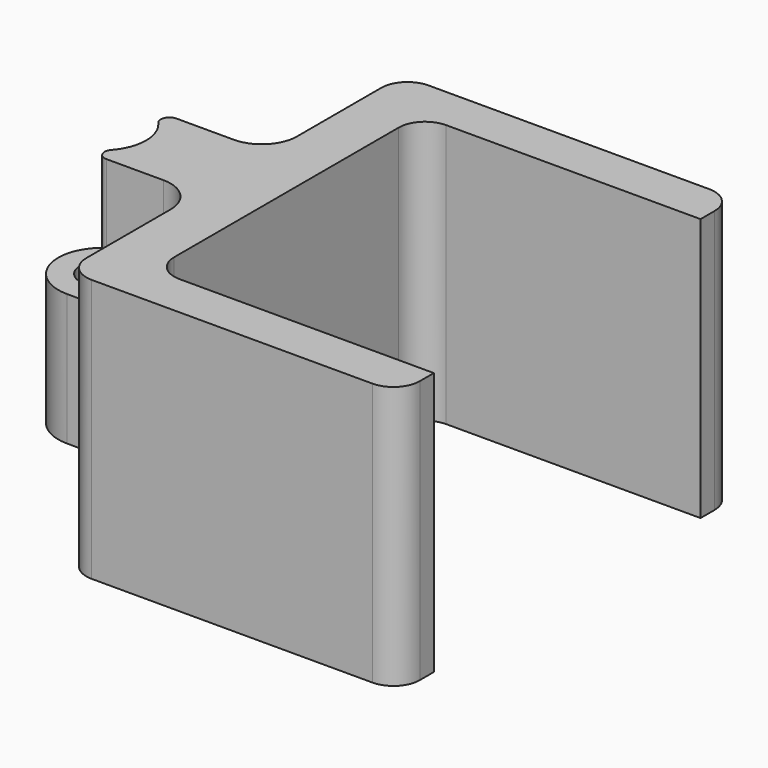
from build123d import *

# Parameters (mm, degrees)
F1_DEPTH    = 30
F2_DEPTH    = 30
F3_DEPTH    = 15
F4_R        = 2.5
F5_DEPTH    = 25
F6_R        = 3
F7_R        = 4
F8_T1_DEPTH = 26.1803398875
F9_SIZE     = 1


# Not quite as in the source:
# - a fillet or chamfer that OpenCascade refuses, or shapes differently, is made with other operations: its cross-section is extruded or revolved along the edge and cut away or added


with BuildPart() as f1:
    # F0 (on Top) → F1 (new body)
    with BuildSketch(Plane.XY):
        with BuildLine():
            ThreePointArc((-71.5824067593, 19.101677686), (-68.0468728533, 17.6372115919), (-66.5824067593, 14.101677686))
            ThreePointArc((-66.5824067593, 14.101677686), (-68.0468728533, 10.56614378), (-71.5824067593, 9.101677686))
            Line((-71.5824067593, 9.101677686), (-56.5824067593, 9.101677686))
            Line((-56.5824067593, 9.101677686), (-56.5824067593, 19.101677686))
            Line((-56.5824067593, 19.101677686), (-71.5824067593, 19.101677686))
        make_face()
    extrude(amount=F1_DEPTH)

    # F0 (on Top) → F2 (join)
    with BuildSketch(Plane.XY):
        Polygon((-56.5824067593, 38.101677686), (-56.5824067593, 33.101677686), (-50.5824067593, 33.101677686), (-18.5824067593, 33.101677686), (-18.5824067593, 38.101677686), align=None)
        Polygon((-56.5824067593, 33.101677686), (-56.5824067593, 19.101677686), (-56.5824067593, 9.101677686), (-56.5824067593, -4.898322314), (-50.5824067593, -4.898322314), (-50.5824067593, 33.101677686), align=None)
        Polygon((-50.5824067593, -4.898322314), (-56.5824067593, -4.898322314), (-56.5824067593, -9.898322314), (-18.5824067593, -9.898322314), (-18.5824067593, -4.898322314), align=None)
    extrude(amount=F2_DEPTH)

    # F0 (on Top) → F3 (join)
    with BuildSketch(Plane.XY):
        with BuildLine():
            ThreePointArc((-71.5824067593, 9.101677686), (-68.0468728533, 10.56614378), (-66.5824067593, 14.101677686))
            ThreePointArc((-66.5824067593, 14.101677686), (-68.0468728533, 17.6372115919), (-71.5824067593, 19.101677686))
            Line((-71.5824067593, 19.101677686), (-71.5824067593, 9.101677686))
        make_face()
        with BuildLine():
            Line((-71.5824067593, 9.101677686), (-71.5824067593, 19.101677686))
            ThreePointArc((-71.5824067593, 19.101677686), (-76.5824067593, 14.101677686), (-71.5824067593, 9.101677686))
        make_face()
    extrude(amount=F3_DEPTH)

    # F4 (on face) → F5 (cut)
    with BuildSketch(Plane.XY.offset(15)):
        with Locations((-71.5824067593, 14.101677686)):
            Circle(F4_R)
    extrude(amount=-F5_DEPTH, mode=Mode.SUBTRACT)

    # F6
    f6_edges = [f1.edges().sort_by_distance(p)[0] for p in [
        (-18.582407, -9.898322, 15),
        (-18.582407, 38.101678, 15),
        (-50.582407, 33.101678, 15),
        (-50.582407, -4.898322, 15),
        (-56.582407, -9.898322, 15),
        (-56.582407, 38.101678, 15),
    ]]
    fillet(f6_edges, radius=F6_R)

    # F7
    f7_edges = [f1.edges().sort_by_distance(p)[0] for p in [
        (-56.582407, 9.101678, 15),
        (-56.582407, 19.101678, 15),
    ]]
    fillet(f7_edges, radius=F7_R)

    # F8: fillet of radius 1 on 4 edges, made by hand

    # F8_s2 → F8_t1 (cut)
    with BuildSketch(Plane.XY.offset(15)):
        with BuildLine():
            ThreePointArc((-67.1102708043, 19.101677686), (-68.0231417334, 18.5099259764), (-67.8556267968, 17.4350110193))
            ThreePointArc((-67.8556267968, 17.4350110193), (-69.5411653069, 18.6660323319), (-71.5824067593, 19.101677686))
            Line((-71.5824067593, 19.101677686), (-67.1102708043, 19.101677686))
        make_face()
        with BuildLine():
            ThreePointArc((-67.1102708043, 9.101677686), (-68.0231417334, 9.6934293955), (-67.8556267968, 10.7683443526))
            ThreePointArc((-67.8556267968, 10.7683443526), (-69.5411653069, 9.5373230401), (-71.5824067593, 9.101677686))
            Line((-71.5824067593, 9.101677686), (-67.1102708043, 9.101677686))
        make_face()
    extrude(amount=F8_T1_DEPTH, mode=Mode.SUBTRACT)

    # F9
    f9_edges = [f1.edges().sort_by_distance(p)[0] for p in [
        (-74.082407, 14.101678, 0),
    ]]
    chamfer(f9_edges, length=F9_SIZE)


solid = f1.part
